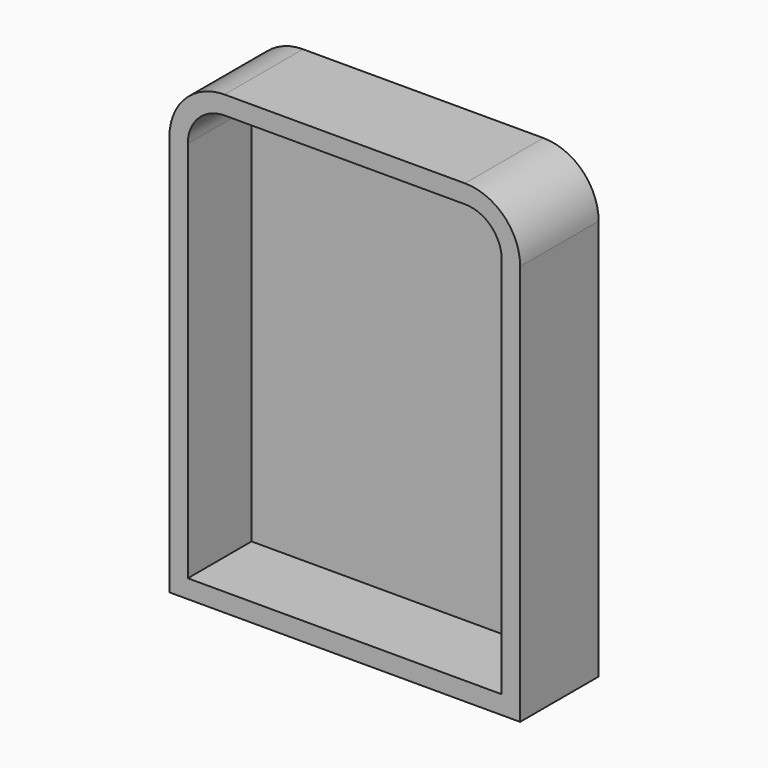
from build123d import *

# Parameters (mm, degrees)
F1_DEPTH = 8
F2_DEPTH = 1.5


# Not quite as in the source:
# - a feature names something its author has since deleted; it is built from what else it names


with BuildPart() as f1:
    # F0 (on Front) → F1 (new body)
    with BuildSketch(Plane.XZ):
        with BuildLine():
            Line((-27.1, 31.2), (-27.1, -1.5))
            Line((-27.1, -1.5), (1.5, -1.5))
            Line((1.5, -1.5), (1.5, 31.2))
            ThreePointArc((1.5, 31.2), (0.1819805153, 34.3819805153), (-3, 35.7))
            Line((-3, 35.7), (-22.6, 35.7))
            ThreePointArc((-22.6, 35.7), (-25.7819805153, 34.3819805153), (-27.1, 31.2))
        make_face()
        with BuildLine():
            ThreePointArc((-25.6, 31.2), (-24.7213203436, 33.3213203436), (-22.6, 34.2))
            Line((-22.6, 34.2), (-3, 34.2))
            ThreePointArc((-3, 34.2), (-0.8786796564, 33.3213203436), (0, 31.2))
            Line((0, 31.2), (0, 0))
            Line((0, 0), (-25.6, 0))
            Line((-25.6, 0), (-25.6, 31.2))
        make_face(mode=Mode.SUBTRACT)
    extrude(amount=F1_DEPTH)

    # F0 (on Front) → F2 (join)
    with BuildSketch(Plane.XZ):
        with BuildLine():
            Line((-3, 34.2), (-22.6, 34.2))
            ThreePointArc((-22.6, 34.2), (-24.7213203436, 33.3213203436), (-25.6, 31.2))
            Line((-25.6, 31.2), (-25.6, 0))
            Line((-25.6, 0), (0, 0))
            Line((0, 0), (0, 31.2))
            ThreePointArc((0, 31.2), (-0.8786796564, 33.3213203436), (-3, 34.2))
        make_face()
    extrude(amount=F2_DEPTH)


solid = f1.part
